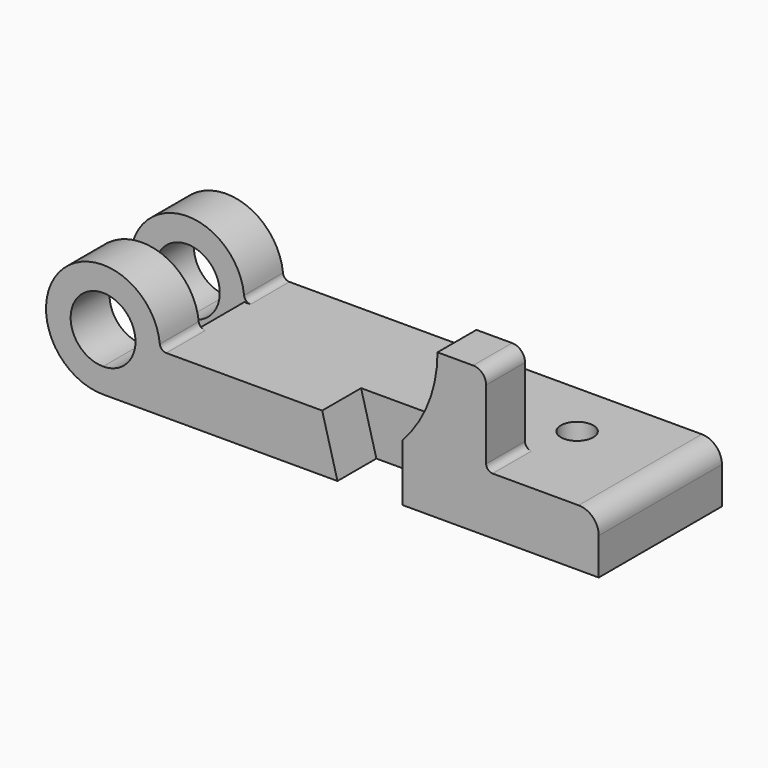
from build123d import *

# Parameters (mm, degrees)
F1_DEPTH = 60.325
F2_DEPTH = 19.05
F0_W     = 19.05
F0_H     = 34.798
F3_DEPTH = 19.05
F4_DEPTH = 19.05
F8_R     = 6.35
F9_DEPTH = 25.4
F10_R    = 7.874
F11_R    = 5.08
F12_R    = 2.54


with BuildPart() as f1:
    # F0 (on Front) → F1 (new body)
    with BuildSketch(Plane.XZ):
        with BuildLine():
            ThreePointArc((-38.3635606445, 0), (-44.9103098714, -15.8052507731), (-60.7155606445, -22.352))
            Line((-60.7155606445, -22.352), (31.1308393555, -22.352))
            Line((31.1308393555, -22.352), (25.1364393555, 0))
            Line((25.1364393555, 0), (-38.3635606445, 0))
        make_face()
        Polygon((25.1364393555, 0), (31.1308393555, -22.352), (56.5308393555, -22.352), (56.5308393555, 0), align=None)
        Polygon((56.5308393555, 0), (56.5308393555, -22.352), (133.4928393555, -22.352), (133.4928393555, 0), (89.3730393555, 0), (70.3230393555, 0), align=None)
    extrude(amount=-F1_DEPTH)

    # F0 (on Front) → F2 (cut)
    with BuildSketch(Plane.XZ):
        Polygon((25.1364393555, 0), (31.1308393555, -22.352), (56.5308393555, -22.352), (56.5308393555, 0), align=None)
    extrude(amount=-F2_DEPTH, mode=Mode.SUBTRACT)

    # F0 (on Front) → F3 (join)
    with BuildSketch(Plane.XZ):
        with BuildLine():
            ThreePointArc((70.3230393555, 34.798), (66.7492677026, 16.0821939471), (56.5308393555, 0))
            Line((56.5308393555, 0), (70.3230393555, 0))
            Line((70.3230393555, 0), (70.3230393555, 34.798))
        make_face()
        with Locations((79.8480393555, 17.399)):
            Rectangle(F0_W, F0_H)
    extrude(amount=-F3_DEPTH)


with BuildPart() as f4:
    # F0 (on Front) → F4 (new body)
    with BuildSketch(Plane.XZ):
        with BuildLine():
            ThreePointArc((-38.3635606445, 0), (-76.5208114176, 15.8052507731), (-60.7155606445, -22.352))
            ThreePointArc((-60.7155606445, -22.352), (-44.9103098714, -15.8052507731), (-38.3635606445, 0))
        make_face()
        with BuildLine():
            ThreePointArc((-60.7155606445, -12.7), (-69.6958167656, 8.9802561211), (-48.0155606445, 0))
            ThreePointArc((-48.0155606445, 0), (-51.7353045234, -8.9802561211), (-60.7155606445, -12.7))
        make_face(mode=Mode.SUBTRACT)
    extrude(amount=-F4_DEPTH)


with BuildPart() as f6_1:
    # F6: instance of F4
    add(f4.part.mirror(Plane.XZ.offset(-30.1625)))


with BuildPart() as f1_1:
    add(f1.part)

    # F7: union F4, F6_1
    add(f4.part)
    add(f6_1.part)

    # F8 (on face) → F9 (cut)
    with BuildSketch(Plane.XY):
        with Locations((94.6308393555, 37.973)):
            Circle(F8_R)
    extrude(amount=-F9_DEPTH, mode=Mode.SUBTRACT)

    # F10
    f10_edges = [f1_1.edges().sort_by_distance(p)[0] for p in [
        (133.492839, 30.1625, 0),
    ]]
    fillet(f10_edges, radius=F10_R)

    # F11
    f11_edges = [f1_1.edges().sort_by_distance(p)[0] for p in [
        (89.373039, 9.525, 34.798),
    ]]
    fillet(f11_edges, radius=F11_R)

    # F12
    f12_edges = [f1_1.edges().sort_by_distance(p)[0] for p in [
        (-38.363561, 50.8, 0),
        (-38.363561, 9.525, 0),
        (89.373039, 9.525, 0),
    ]]
    fillet(f12_edges, radius=F12_R)


solid = f1_1.part
